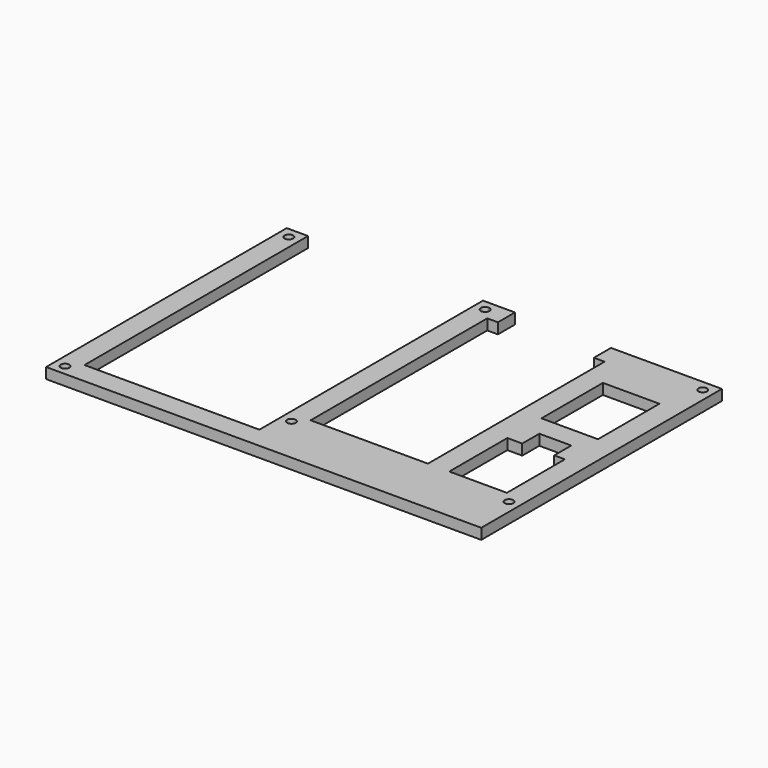
from build123d import *

# Parameters (mm, degrees)
F1_DEPTH = 5


# Not quite as in the source:
# - a feature names something its author has since deleted; it is built from what else it names


with BuildPart() as f1:
    # F0 (on Top) → F1 (new body)
    with BuildSketch(Plane.XY):
        with BuildLine():
            Line((-134.3440142274, -1.256315279), (-139.3440142274, -1.256315279))
            Line((-139.3440142274, -1.256315279), (-139.3440142274, -6.256315279))
            Line((-139.3440142274, -6.256315279), (-136.3440142274, -6.256315279))
            ThreePointArc((-136.3440142274, -6.256315279), (-135.7582277898, -4.8421017166), (-134.3440142274, -4.256315279))
            Line((-134.3440142274, -4.256315279), (-134.3440142274, -1.256315279))
        make_face()
        with BuildLine():
            Line((-129.3440142274, -1.256315279), (-134.3440142274, -1.256315279))
            Line((-134.3440142274, -1.256315279), (-134.3440142274, -4.256315279))
            ThreePointArc((-134.3440142274, -4.256315279), (-132.929800665, -4.8421017166), (-132.3440142274, -6.256315279))
            ThreePointArc((-132.3440142274, -6.256315279), (-134.3440142274, -8.256315279), (-136.3440142274, -6.256315279))
            Line((-136.3440142274, -6.256315279), (-139.3440142274, -6.256315279))
            Line((-139.3440142274, -6.256315279), (-139.3440142274, -11.256315279))
            Line((-139.3440142274, -11.256315279), (-129.3440142274, -11.256315279))
            Line((-129.3440142274, -11.256315279), (-129.3440142274, -1.256315279))
        make_face()
        with BuildLine():
            Line((-221.3440142274, -6.256315279), (-221.3440142274, -1.256315279))
            Line((-221.3440142274, -1.256315279), (-231.3440142274, -1.256315279))
            Line((-231.3440142274, -1.256315279), (-231.3440142274, -132.256315279))
            Line((-231.3440142274, -132.256315279), (-221.3440142274, -132.256315279))
            Line((-221.3440142274, -132.256315279), (-221.3440142274, -128.856315279))
            Line((-221.3440142274, -128.856315279), (-221.3440142274, -14.656315279))
            Line((-221.3440142274, -14.656315279), (-221.3440142274, -11.256315279))
            Line((-221.3440142274, -11.256315279), (-226.3440142274, -11.256315279))
            Line((-226.3440142274, -11.256315279), (-226.3440142274, -8.256315279))
            ThreePointArc((-226.3440142274, -8.256315279), (-227.7582277898, -4.8421017166), (-224.3440142274, -6.256315279))
            Line((-224.3440142274, -6.256315279), (-221.3440142274, -6.256315279))
        make_face()
        Polygon((-124.3440142274, -1.256315279), (-129.3440142274, -1.256315279), (-129.3440142274, -11.256315279), (-126.5440142274, -11.256315279), (-126.3440142274, -11.256315279), (-124.3440142274, -11.256315279), align=None)
        Polygon((-129.3440142274, -11.256315279), (-139.3440142274, -11.256315279), (-139.3440142274, -14.656315279), (-139.3440142274, -114.756315279), (-129.3440142274, -114.756315279), (-129.3440142274, -111.756315279), (-129.3440142274, -108.756315279), (-129.3440142274, -27.956315279), (-129.3440142274, -27.456315279), (-129.3440142274, -14.056315279), align=None)
        with BuildLine():
            Line((-221.3440142274, -11.256315279), (-221.3440142274, -6.256315279))
            Line((-221.3440142274, -6.256315279), (-224.3440142274, -6.256315279))
            ThreePointArc((-224.3440142274, -6.256315279), (-224.929800665, -7.6705288414), (-226.3440142274, -8.256315279))
            Line((-226.3440142274, -8.256315279), (-226.3440142274, -11.256315279))
            Line((-226.3440142274, -11.256315279), (-221.3440142274, -11.256315279))
        make_face()
        with BuildLine():
            Line((-221.3440142274, -132.256315279), (-231.3440142274, -132.256315279))
            Line((-231.3440142274, -132.256315279), (-231.3440142274, -137.3912245035))
            Line((-231.3440142274, -137.3912245035), (-228.3440142274, -137.3912245035))
            ThreePointArc((-228.3440142274, -137.3912245035), (-226.3440142274, -135.3912245035), (-224.3440142274, -137.3912245035))
            ThreePointArc((-224.3440142274, -137.3912245035), (-224.929800665, -138.8054380659), (-226.3440142274, -139.3912245035))
            Line((-226.3440142274, -139.3912245035), (-226.3440142274, -142.256315279))
            Line((-226.3440142274, -142.256315279), (-221.3440142274, -142.256315279))
            Line((-221.3440142274, -142.256315279), (-221.3440142274, -132.256315279))
        make_face()
        with BuildLine():
            Line((-129.3440142274, -114.756315279), (-139.3440142274, -114.756315279))
            Line((-139.3440142274, -114.756315279), (-139.3440142274, -119.756315279))
            Line((-139.3440142274, -119.756315279), (-136.3440142274, -119.756315279))
            ThreePointArc((-136.3440142274, -119.756315279), (-134.3440142274, -117.756315279), (-132.3440142274, -119.756315279))
            ThreePointArc((-132.3440142274, -119.756315279), (-132.929800665, -121.1705288414), (-134.3440142274, -121.756315279))
            Line((-134.3440142274, -121.756315279), (-134.3440142274, -124.756315279))
            Line((-134.3440142274, -124.756315279), (-129.3440142274, -124.756315279))
            Line((-129.3440142274, -124.756315279), (-129.3440142274, -114.756315279))
        make_face()
        Polygon((-217.9440142274, -132.256315279), (-221.3440142274, -132.256315279), (-221.3440142274, -142.256315279), (-139.3440142274, -142.256315279), (-139.4949736476, -132.256315279), (-142.7440142274, -132.256315279), (-147.4240142274, -132.256315279), (-151.4240142274, -132.256315279), align=None)
        with BuildLine():
            Line((-228.3440142274, -137.3912245035), (-231.3440142274, -137.3912245035))
            Line((-231.3440142274, -137.3912245035), (-231.3440142274, -142.256315279))
            Line((-231.3440142274, -142.256315279), (-226.3440142274, -142.256315279))
            Line((-226.3440142274, -142.256315279), (-226.3440142274, -139.3912245035))
            ThreePointArc((-226.3440142274, -139.3912245035), (-227.7582277898, -138.8054380659), (-228.3440142274, -137.3912245035))
        make_face()
        with BuildLine():
            Line((-79.3440142274, -1.256315279), (-79.3440142274, -11.256315279))
            Line((-79.3440142274, -11.256315279), (-77.3440142274, -11.256315279))
            Line((-77.3440142274, -11.256315279), (-74.3440142274, -11.256315279))
            Line((-74.3440142274, -11.256315279), (-32.3440142274, -11.256315279))
            Line((-32.3440142274, -11.256315279), (-32.3440142274, -8.256315279))
            ThreePointArc((-32.3440142274, -8.256315279), (-33.7582277898, -4.8421017166), (-30.3440142274, -6.256315279))
            Line((-30.3440142274, -6.256315279), (-27.3440142274, -6.256315279))
            Line((-27.3440142274, -6.256315279), (-27.3440142274, -1.256315279))
            Line((-27.3440142274, -1.256315279), (-79.3440142274, -1.256315279))
        make_face()
        Polygon((-126.3440142274, -114.756315279), (-129.3440142274, -114.756315279), (-129.3440142274, -124.756315279), (-74.3440142274, -124.756315279), (-74.3440142274, -114.756315279), (-77.1940142274, -114.756315279), (-77.3440142274, -114.756315279), align=None)
        with BuildLine():
            Line((-136.3440142274, -119.756315279), (-139.3440142274, -119.756315279))
            Line((-139.3440142274, -119.756315279), (-139.3440142274, -124.756315279))
            Line((-139.3440142274, -124.756315279), (-139.1930548072, -124.756315279))
            Line((-139.1930548072, -124.756315279), (-134.3440142274, -124.756315279))
            Line((-134.3440142274, -124.756315279), (-134.3440142274, -121.756315279))
            ThreePointArc((-134.3440142274, -121.756315279), (-135.7582277898, -121.1705288414), (-136.3440142274, -119.756315279))
        make_face()
        Polygon((-139.3440142274, -132.256315279), (-139.4949736476, -132.256315279), (-139.3440142274, -142.256315279), (-129.3440142274, -142.256315279), (-129.3440142274, -124.756315279), (-134.3440142274, -124.756315279), (-139.1930548072, -124.756315279), (-139.3440142274, -124.756315279), (-139.3440142274, -128.856315279), align=None)
        Polygon((-74.3440142274, -124.756315279), (-129.3440142274, -124.756315279), (-129.3440142274, -142.256315279), (-77.3440142274, -142.256315279), (-74.3440142274, -142.256315279), align=None)
        Polygon((-32.3440142274, -11.256315279), (-74.3440142274, -11.256315279), (-74.3440142274, -14.256315279), (-74.3440142274, -26.056315279), (-74.3440142274, -103.156315279), (-74.3440142274, -111.906315279), (-74.3440142274, -114.756315279), (-64.3440142274, -114.756315279), (-64.3440142274, -105.506315279), (-64.3440142274, -82.706315279), (-64.3440142274, -80.756315279), (-64.3440142274, -60.756315279), (-64.3440142274, -59.006315279), (-64.3440142274, -26.456315279), (-64.3440142274, -24.756315279), (-62.6440142274, -24.756315279), (-39.5440142274, -24.756315279), (-37.8440142274, -24.756315279), (-27.3440142274, -24.756315279), (-27.3440142274, -14.656315279), (-27.3440142274, -11.256315279), align=None)
        with BuildLine():
            Line((-27.3440142274, -11.256315279), (-27.3440142274, -6.256315279))
            Line((-27.3440142274, -6.256315279), (-30.3440142274, -6.256315279))
            ThreePointArc((-30.3440142274, -6.256315279), (-30.929800665, -7.6705288414), (-32.3440142274, -8.256315279))
            Line((-32.3440142274, -8.256315279), (-32.3440142274, -11.256315279))
            Line((-32.3440142274, -11.256315279), (-27.3440142274, -11.256315279))
        make_face()
        Polygon((-74.3440142274, -114.756315279), (-74.3440142274, -124.756315279), (-37.3440142274, -124.756315279), (-37.3440142274, -119.756315279), (-37.3440142274, -114.756315279), (-39.2940142274, -114.756315279), (-62.3940142274, -114.756315279), (-64.3440142274, -114.756315279), align=None)
        Polygon((-37.3440142274, -124.756315279), (-74.3440142274, -124.756315279), (-74.3440142274, -142.256315279), (-27.3440142274, -142.256315279), (-27.3440142274, -124.756315279), (-32.3440142274, -124.756315279), align=None)
        with BuildLine():
            Line((-37.3440142274, -119.756315279), (-37.3440142274, -124.756315279))
            Line((-37.3440142274, -124.756315279), (-32.3440142274, -124.756315279))
            Line((-32.3440142274, -124.756315279), (-32.3440142274, -121.756315279))
            ThreePointArc((-32.3440142274, -121.756315279), (-33.7582277898, -121.1705288414), (-34.3440142274, -119.756315279))
            Line((-34.3440142274, -119.756315279), (-37.3440142274, -119.756315279))
        make_face()
        with BuildLine():
            Line((-32.3440142274, -121.756315279), (-32.3440142274, -124.756315279))
            Line((-32.3440142274, -124.756315279), (-27.3440142274, -124.756315279))
            Line((-27.3440142274, -124.756315279), (-27.3440142274, -114.756315279))
            Line((-27.3440142274, -114.756315279), (-37.3440142274, -114.756315279))
            Line((-37.3440142274, -114.756315279), (-37.3440142274, -119.756315279))
            Line((-37.3440142274, -119.756315279), (-34.3440142274, -119.756315279))
            ThreePointArc((-34.3440142274, -119.756315279), (-32.3440142274, -117.756315279), (-30.3440142274, -119.756315279))
            ThreePointArc((-30.3440142274, -119.756315279), (-30.929800665, -121.1705288414), (-32.3440142274, -121.756315279))
        make_face()
        Polygon((-27.3440142274, -114.756315279), (-27.3440142274, -24.756315279), (-37.8440142274, -24.756315279), (-37.8440142274, -26.456315279), (-37.8440142274, -59.006315279), (-37.8440142274, -60.756315279), (-39.5940142274, -60.756315279), (-62.5940142274, -60.756315279), (-64.3440142274, -60.756315279), (-64.3440142274, -80.756315279), (-62.3940142274, -80.756315279), (-57.3440142274, -80.756315279), (-57.3440142274, -70.756315279), (-42.3440142274, -70.756315279), (-42.3440142274, -80.756315279), (-39.2940142274, -80.756315279), (-37.3440142274, -80.756315279), (-37.3440142274, -82.706315279), (-37.3440142274, -105.506315279), (-37.3440142274, -114.756315279), align=None)
    extrude(amount=F1_DEPTH)


solid = f1.part
